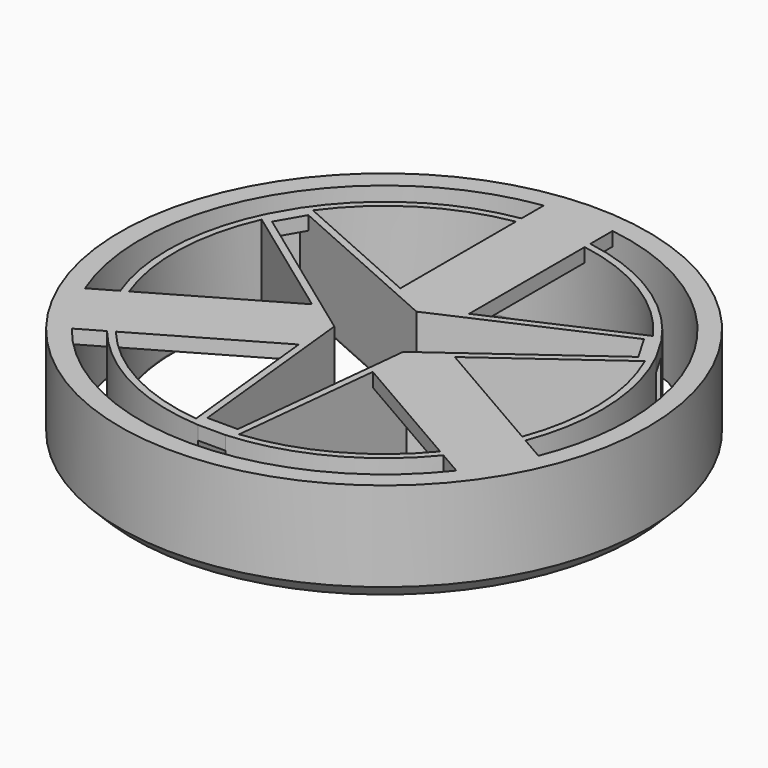
from build123d import *

# Parameters (mm, degrees)
F0_R      = 36.5
F1_DEPTH  = 20
F2_R      = 35.5
F2_R_2    = 31.5
F3_DEPTH  = 20.001
F5_DEPTH  = 20.001
F8_DEPTH  = 20.001
F10_COUNT = 3
F11_R     = 32.9719695727
F12_DEPTH = 2
F13_R     = 36.5
F14_DEPTH = 5
F15_R     = 0.49999
F16_R     = 38.3472414885
F16_R_2   = 36.3472414885
F17_DEPTH = 20
F18_SIZE  = 1.99999
F19_R     = 41.0530040579
F20_DEPTH = 5
F22_DEPTH = 2


# Not quite as in the source:
# - a fillet or chamfer is up to 0.001 mm smaller than in the source, because OpenCascade refuses the exact size


with BuildPart() as f1:
    # F0 (on Top) → F1 (new body)
    with BuildSketch(Plane.XY):
        Circle(F0_R)
    extrude(amount=F1_DEPTH)

    # F2 (on face) → F3 (cut, through all)
    with BuildSketch(Plane(origin=(0, 0, 0), x_dir=(1, 0, 0), z_dir=(0, 0, -1))):
        Circle(F2_R)
        Circle(F2_R_2, mode=Mode.SUBTRACT)
    extrude(amount=-F3_DEPTH, mode=Mode.SUBTRACT)

    # F4 (on face) → F5 (cut, through all)
    with BuildSketch(Plane(origin=(0, 0, 0), x_dir=(1, 0, 0), z_dir=(0, 0, -1))):
        with BuildLine():
            Line((-5, 2.8867513459), (0, 0))
            Line((0, 0), (0, 31.5))
            ThreePointArc((0, 31.5), (-1, 31.4841229829), (-1.9989919354, 31.4365079365))
            Line((-1.9989919354, 31.4365079365), (-5, 2.8867513459))
        make_face()
        with BuildLine():
            Line((0, 31.5), (0, 0))
            Line((0, 0), (27.2798002192, -15.75))
            ThreePointArc((27.2798002192, -15.75), (27.766050319, -14.8760360876), (28.224310447, -13.9870761702))
            Line((28.224310447, -13.9870761702), (5, 2.8867513459))
            Line((5, 2.8867513459), (1.9989919354, 31.4365079365))
            ThreePointArc((1.9989919354, 31.4365079365), (1, 31.4841229829), (0, 31.5))
        make_face()
        with BuildLine():
            Line((-27.2798002192, -15.75), (0, 0))
            Line((0, 0), (-5, 2.8867513459))
            Line((-5, 2.8867513459), (-28.224310447, -13.9870761702))
            ThreePointArc((-28.224310447, -13.9870761702), (-27.766050319, -14.8760360876), (-27.2798002192, -15.75))
        make_face()
        with BuildLine():
            Line((27.2798002192, -15.75), (0, 0))
            Line((0, 0), (-27.2798002192, -15.75))
            ThreePointArc((-27.2798002192, -15.75), (-26.766050319, -16.6080868952), (-26.2253185116, -17.4494317663))
            Line((-26.2253185116, -17.4494317663), (0, -5.7735026919))
            Line((0, -5.7735026919), (26.2253185116, -17.4494317663))
            ThreePointArc((26.2253185116, -17.4494317663), (26.766050319, -16.6080868952), (27.2798002192, -15.75))
        make_face()
    extrude(amount=-F5_DEPTH, mode=Mode.SUBTRACT)

    # F7 (on face) → F8 (cut, through all)
    with BuildSketch(Plane(origin=(0, 0, 0), x_dir=(1, 0, 0), z_dir=(0, 0, -1))):
        with BuildLine():
            Line((-5.9479783255, 3.4340668874), (-3.119758175, 30.340024867))
            ThreePointArc((-3.119758175, 30.340024867), (-26.4137748154, 15.25), (-27.8351113737, -12.4682226003))
            Line((-27.8351113737, -12.4682226003), (-5.9479783255, 3.4340668874))
        make_face()
        Polygon((0, 33.3932489157), (0, 0), (-27.0690638572, -15.5309122056), (-27.0690638572, -19.8186486959), (-19.1532429308, -28.0642919242), (-5.5204438977, -33.4514454007), (14.1841255464, -31.0257077197), (26.5826005489, -22.0174863935), (32.7393487096, -5.7460800745), (32.7393487096, 6.6773579456), (25.4831798375, 23.2785902917), (10.75096149, 31.7441187799), align=None)
    extrude(amount=-F8_DEPTH, mode=Mode.SUBTRACT)


with BuildPart() as f10_1:
    # F10: instance of F1
    add(f1.part.rotate(Axis((0, 0, 8.8435821235), (0, 0, 1)), 1 * 360 / F10_COUNT))


with BuildPart() as f10_2:
    # F10: instance of F1
    add(f1.part.rotate(Axis((0, 0, 8.8435821235), (0, 0, 1)), 2 * 360 / F10_COUNT))


with BuildPart() as f12_tool:
    # F11 (on Top) → F12 (new body)
    with BuildSketch(Plane.XY):
        Circle(F11_R)
    extrude(amount=F12_DEPTH)


with BuildPart() as f1_1:
    add(f1.part)

    # F12: cut by f12_tool
    add(f12_tool.part, mode=Mode.SUBTRACT)



with BuildPart() as f10_1_1:
    add(f10_1.part)

    # F12: cut by f12_tool
    add(f12_tool.part, mode=Mode.SUBTRACT)


with BuildPart() as f10_2_1:
    add(f10_2.part)

    # F12: cut by f12_tool
    add(f12_tool.part, mode=Mode.SUBTRACT)


with BuildPart() as f1_2:
    add(f1_1.part)

    add(f10_1_1.part)  # F14 merges F10_1

    add(f10_2_1.part)  # F14 merges F10_2
    # F13 (on face) → F14 (join)
    with BuildSketch(Plane.XY.offset(20)):
        Circle(F13_R)
    extrude(amount=-F14_DEPTH)

    # F15 (radius 0.5 in the source; OpenCascade refuses exactly that, so slightly less here)
    f15_edges = [f1_2.edges().sort_by_distance(p)[0] for p in [
        (17.75, 30.743902, 0),
        (18.25, 31.609927, 0),
        (-27.2798, -15.75, 2),
        (-16.612155, 5.550162, 2),
        (-3.499496, -17.16163, 2),
        (-26.413775, -15.25, 2),
        (-4.533868, -16.887046, 2),
        (-16.891545, 4.517078, 2),
        (0, 31.5, 2),
        (13.112659, 11.611467, 2),
        (-13.112659, 11.611467, 2),
        (0, 30.5, 2),
        (-12.357677, 12.369968, 2),
        (12.357677, 12.369968, 2),
        (27.2798, -15.75, 2),
        (3.499496, -17.16163, 2),
        (16.612155, 5.550162, 2),
        (26.413775, -15.25, 2),
        (16.891545, 4.517078, 2),
        (4.533868, -16.887046, 2),
    ]]
    fillet(f15_edges, radius=F15_R)

    # F16 (on Top) → F17 (join)
    with BuildSketch(Plane.XY):
        with Locations((-0.1366314536, 0.0683155085)):
            Circle(F16_R)
        with Locations((-0.1366314536, 0.0683155085)):
            Circle(F16_R_2, mode=Mode.SUBTRACT)
    extrude(amount=F17_DEPTH)

    # F18 (size 2 in the source; OpenCascade refuses exactly that, so slightly less here)
    f18_edges = [f1_2.edges().sort_by_distance(p)[0] for p in [
        (-38.483873, 0.068316, 0),
    ]]
    chamfer(f18_edges, length=F18_SIZE)

    # F19 (on face) → F20 (cut)
    with BuildSketch(Plane.XY.offset(20)):
        Circle(F19_R)
    extrude(amount=-F20_DEPTH, mode=Mode.SUBTRACT)

    # F21 (on face) → F22 (join)
    with BuildSketch(Plane.XY.offset(15)):
        Polygon((-28.6765527518, -22.3299181426), (-4.4278414458, -8.3299181426), (-5, -2.8867513459), (-9.4278414458, 0.3303358953), (-33.6765527518, -13.6696641047), (-31.1765527518, -17.9997911236), align=None)
        Polygon((4.4278414458, -8.3299181426), (28.6765527518, -22.3299181426), (31.1765527518, -17.9997911236), (33.6765527518, -13.6696641047), (9.4278414458, 0.3303358953), (5, -2.8867513459), align=None)
        Polygon((5, 7.9995822473), (5, 35.9995822473), (0, 35.9995822473), (-5, 35.9995822473), (-5, 7.9995822473), (0, 5.7735026919), align=None)
        Polygon((-26.2253185116, 17.4494317663), (-28.224310447, 13.9870761702), (-26.5973746535, 12.8050116253), (-24.38815269, 16.6314963112), align=None)
        Polygon((2.2092219635, -29.4365079365), (-2.2092219635, -29.4365079365), (-1.9989919354, -31.4365079365), (1.9989919354, -31.4365079365), align=None)
        Polygon((24.38815269, 16.6314963112), (26.5973746535, 12.8050116253), (28.224310447, 13.9870761702), (26.2253185116, 17.4494317663), align=None)
    extrude(amount=-F22_DEPTH)


solid = f1_2.part
